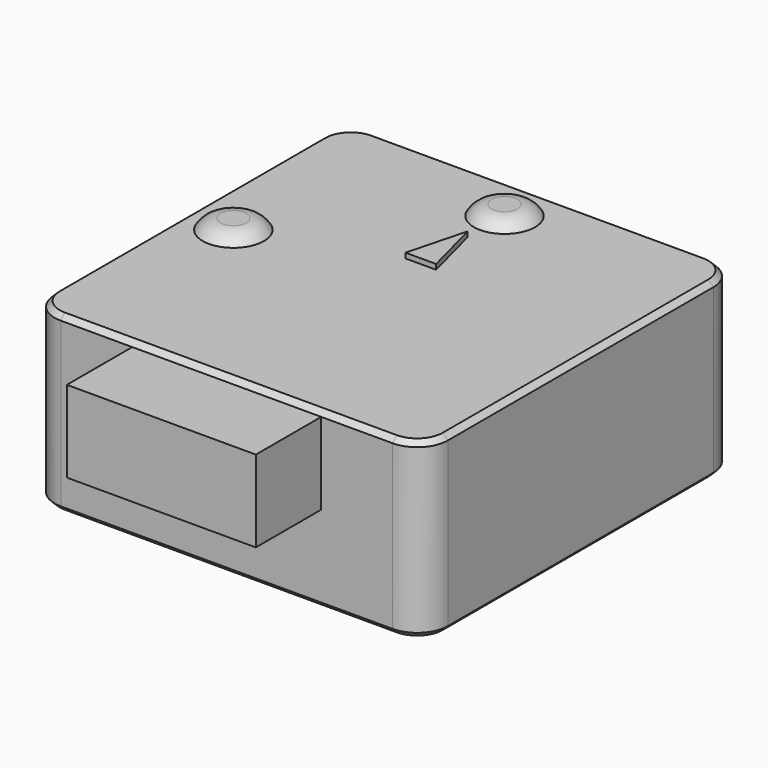
from build123d import *

# Parameters (mm, degrees)
F1_DEPTH = 17
F3_DEPTH = 0.5
F4_DEPTH = 18
F6_R     = 3
F7_SIZE  = 0.5
F8_W     = 18.5
F8_H     = 8
F9_DEPTH = 8


# Not quite as in the source:
# - a fillet or chamfer that OpenCascade refuses, or shapes differently, is made with other operations: its cross-section is extruded or revolved along the edge and cut away or added


with BuildPart() as f1:
    # F0 (on Top) → F1 (new body)
    with BuildSketch(Plane.XY):
        Polygon((-19.25, -19.25), (19.25, -19.25), (19.25, 19.25), (0, 19.25), (-19.25, 19.25), (-19.25, 0), align=None)
        with BuildLine():
            ThreePointArc((-11.75, 0), (-14.75, -3), (-17.75, 0))
            ThreePointArc((-17.75, 0), (-14.75, 3), (-11.75, 0))
        make_face(mode=Mode.SUBTRACT)
        with BuildLine():
            ThreePointArc((3, 14.75), (-2.1213203436, 12.6286796564), (0, 17.75))
            ThreePointArc((0, 17.75), (2.1213203436, 16.8713203436), (3, 14.75))
        make_face(mode=Mode.SUBTRACT)
        with BuildLine():
            ThreePointArc((-11.75, 0), (-14.75, 3), (-17.75, 0))
            ThreePointArc((-17.75, 0), (-14.75, -3), (-11.75, 0))
        make_face()
        with BuildLine():
            ThreePointArc((3, 14.75), (2.1213203436, 16.8713203436), (0, 17.75))
            ThreePointArc((0, 17.75), (-2.1213203436, 12.6286796564), (3, 14.75))
        make_face()
    extrude(amount=F1_DEPTH)

    # F2 (on face) → F3 (join)
    with BuildSketch(Plane.XY.offset(17)):
        Polygon((-1.5, 4.5069497171), (1.5, 4.5069497171), (0, 10.2327093482), align=None)
    extrude(amount=F3_DEPTH)

    # F0 (on Top) → F4 (join)
    with BuildSketch(Plane.XY):
        with BuildLine():
            ThreePointArc((3, 14.75), (2.1213203436, 16.8713203436), (0, 17.75))
            ThreePointArc((0, 17.75), (-2.1213203436, 12.6286796564), (3, 14.75))
        make_face()
        with BuildLine():
            ThreePointArc((-11.75, 0), (-14.75, 3), (-17.75, 0))
            ThreePointArc((-17.75, 0), (-14.75, -3), (-11.75, 0))
        make_face()
    extrude(amount=F4_DEPTH)

    # F5: fillet of radius 2 on 2 edges, made by hand

    # F5_s1 → F5_t2 (revolve, cut)
    with BuildSketch(Plane.YZ):
        with BuildLine():
            ThreePointArc((17.75, 17), (17.0179491924, 17.7320508076), (16.0179491924, 18))
            Line((16.0179491924, 18), (17.75, 18))
            Line((17.75, 18), (17.75, 17))
        make_face()
    revolve(axis=Axis((0, 14.75, 18), (0, 0, 1)), mode=Mode.SUBTRACT)

    # F5_s3 → F5_t4 (revolve, cut)
    with BuildSketch(Plane.XZ):
        with BuildLine():
            ThreePointArc((-17.75, 17), (-17.0179491924, 17.7320508076), (-16.0179491924, 18))
            Line((-16.0179491924, 18), (-17.75, 18))
            Line((-17.75, 18), (-17.75, 17))
        make_face()
    revolve(axis=Axis((-14.75, 0, 18), (0, 0, 1)), mode=Mode.SUBTRACT)

    # F6
    f6_edges = [f1.edges().sort_by_distance(p)[0] for p in [
        (19.25, -19.25, 8.5),
        (-19.25, -19.25, 8.5),
        (-19.25, 19.25, 8.5),
        (19.25, 19.25, 8.5),
    ]]
    fillet(f6_edges, radius=F6_R)

    # F7
    f7_edges = [f1.edges().sort_by_distance(p)[0] for p in [
        (0, 19.25, 17),
        (18.37132, 18.37132, 17),
        (19.25, 0, 17),
        (18.37132, -18.37132, 17),
        (0, -19.25, 17),
        (-18.37132, -18.37132, 17),
        (-19.25, 0, 17),
        (-18.37132, 18.37132, 17),
        (0, -19.25, 0),
        (-18.37132, -18.37132, 0),
        (18.37132, -18.37132, 0),
        (-19.25, 0, 0),
        (19.25, 0, 0),
        (-18.37132, 18.37132, 0),
        (18.37132, 18.37132, 0),
        (0, 19.25, 0),
    ]]
    chamfer(f7_edges, length=F7_SIZE)

    # F8 (on face) → F9 (join)
    with BuildSketch(Plane.XZ.offset(19.25)):
        with Locations((0, 12.5)):
            Rectangle(F8_W, F8_H)
    extrude(amount=F9_DEPTH)


solid = f1.part
